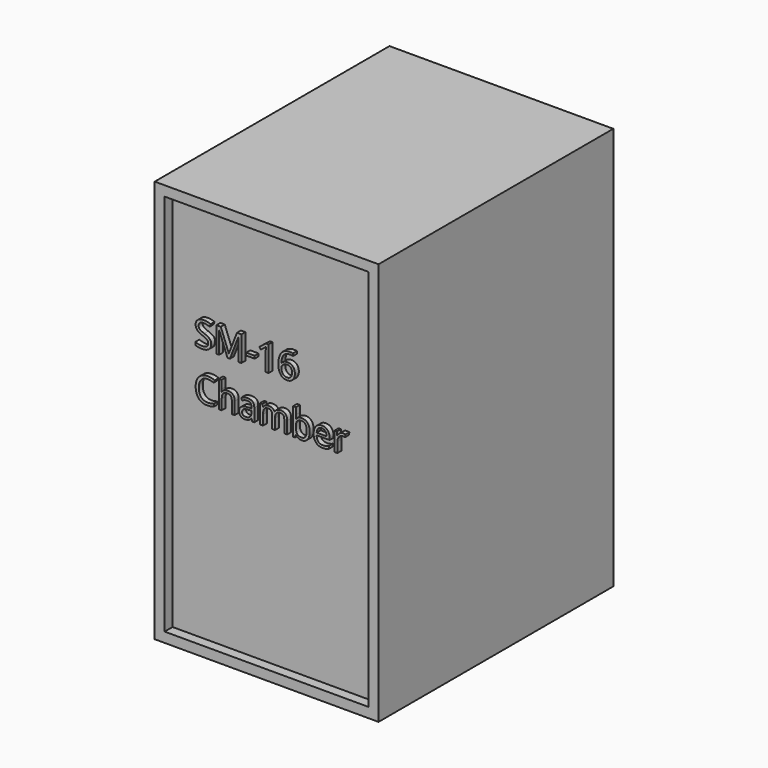
from build123d import *

# Parameters (mm, degrees)
F0_W         = 1143
F0_H         = 1498.6
F1_DEPTH     = 2057.4
F2_W         = 1041.4
F2_H         = 1955.8
F3_DEPTH     = 50.8
F4_TEXT_SIZE = 180.4411343455
F5_DEPTH     = 25.4


# Not quite as in the source:
# - Text() gives the source's letters only with a copy of the font that has no kerning and outlines rounded to 1/6400 em; it was checked with that copy


with BuildPart() as f1:
    # F0 (on Top) → F1 (new body)
    with BuildSketch(Plane.XY):
        Rectangle(F0_W, F0_H)
    extrude(amount=F1_DEPTH)

    # F2 (on face) → F3 (cut)
    with BuildSketch(Plane.XZ.offset(749.3)):
        with Locations((0, 1028.7)):
            Rectangle(F2_W, F2_H)
    extrude(amount=-F3_DEPTH, mode=Mode.SUBTRACT)

    # F4 (on face) → F5 (join)
    with BuildSketch(Plane.XZ.offset(698.5)):
        with Locations((-393.7, 1368.6823832713)):
            Text('SM-16', F4_TEXT_SIZE, font='Open Sans', text_align=(TextAlign.LEFT, TextAlign.BOTTOM))
        with Locations((-393.7, 1123.2824405614)):
            Text('Chamber', F4_TEXT_SIZE, font='Open Sans', text_align=(TextAlign.LEFT, TextAlign.BOTTOM))
    extrude(amount=F5_DEPTH)


solid = f1.part
